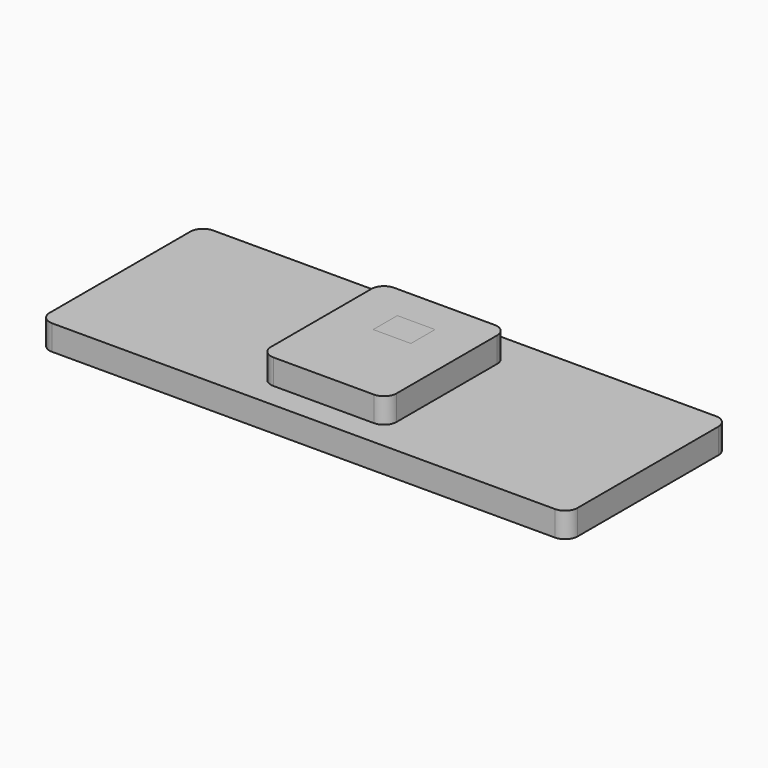
from build123d import *

# Parameters (mm, degrees)
F1_START = 2
F1_DEPTH = 1
F2_DEPTH = 3
F3_START = 2
F0_W     = 1.5
F0_H     = 1.2
F3_DEPTH = 2
F4_START = 3.5
F4_DEPTH = 0.5


# Not quite as in the source:
# - a feature names something its author has since deleted; it is built from what else it names


with BuildPart() as f1:
    # F0 (on Top) → F1 (new body)
    with BuildSketch(Plane.XY.offset(F1_START)):
        with BuildLine():
            Line((10, 4), (-10, 4))
            ThreePointArc((-10, 4), (-10.3535533906, 3.8535533906), (-10.5, 3.5))
            Line((-10.5, 3.5), (-10.5, -3.5))
            ThreePointArc((-10.5, -3.5), (-10.3535533906, -3.8535533906), (-10, -4))
            Line((-10, -4), (10, -4))
            ThreePointArc((10, -4), (10.3535533906, -3.8535533906), (10.5, -3.5))
            Line((10.5, -3.5), (10.5, 3.5))
            ThreePointArc((10.5, 3.5), (10.3535533906, 3.8535533906), (10, 4))
        make_face()
        with BuildLine():
            ThreePointArc((-7.9, 0.5), (-7.7535533906, 0.8535533906), (-7.4, 1))
            Line((-7.4, 1), (-5.9, 1))
            Line((-5.9, 1), (-5.9, -1))
            Line((-5.9, -1), (-7.4, -1))
            ThreePointArc((-7.4, -1), (-7.7535533906, -0.8535533906), (-7.9, -0.5))
            Line((-7.9, -0.5), (-7.9, 0.5))
        make_face(mode=Mode.SUBTRACT)
        with BuildLine():
            Line((-2, 3), (2, 3))
            ThreePointArc((2, 3), (2.3535533906, 2.8535533906), (2.5, 2.5))
            Line((2.5, 2.5), (2.5, -2.5))
            ThreePointArc((2.5, -2.5), (2.3535533906, -2.8535533906), (2, -3))
            Line((2, -3), (-2, -3))
            ThreePointArc((-2, -3), (-2.3535533906, -2.8535533906), (-2.5, -2.5))
            Line((-2.5, -2.5), (-2.5, 2.5))
            ThreePointArc((-2.5, 2.5), (-2.3535533906, 2.8535533906), (-2, 3))
        make_face(mode=Mode.SUBTRACT)
        with BuildLine():
            Line((5.9, -1), (5.9, 1))
            Line((5.9, 1), (7.4, 1))
            ThreePointArc((7.4, 1), (7.7535533906, 0.8535533906), (7.9, 0.5))
            Line((7.9, 0.5), (7.9, -0.5))
            ThreePointArc((7.9, -0.5), (7.7535533906, -0.8535533906), (7.4, -1))
            Line((7.4, -1), (5.9, -1))
        make_face(mode=Mode.SUBTRACT)
    extrude(amount=F1_DEPTH)

    # F0 (on Top) → F2 (join)
    with BuildSketch(Plane.XY):
        with BuildLine():
            Line((-5.9, 1), (-7.4, 1))
            ThreePointArc((-7.4, 1), (-7.7535533906, 0.8535533906), (-7.9, 0.5))
            Line((-7.9, 0.5), (-7.9, -0.5))
            ThreePointArc((-7.9, -0.5), (-7.7535533906, -0.8535533906), (-7.4, -1))
            Line((-7.4, -1), (-5.9, -1))
            Line((-5.9, -1), (-5.9, 1))
        make_face()
        with BuildLine():
            Line((7.4, 1), (5.9, 1))
            Line((5.9, 1), (5.9, -1))
            Line((5.9, -1), (7.4, -1))
            ThreePointArc((7.4, -1), (7.7535533906, -0.8535533906), (7.9, -0.5))
            Line((7.9, -0.5), (7.9, 0.5))
            ThreePointArc((7.9, 0.5), (7.7535533906, 0.8535533906), (7.4, 1))
        make_face()
    extrude(amount=F2_DEPTH)

    # F0 (on Top) → F3 (join)
    with BuildSketch(Plane.XY.offset(F3_START)):
        with BuildLine():
            ThreePointArc((2.5, 2.5), (2.3535533906, 2.8535533906), (2, 3))
            Line((2, 3), (-2, 3))
            ThreePointArc((-2, 3), (-2.3535533906, 2.8535533906), (-2.5, 2.5))
            Line((-2.5, 2.5), (-2.5, -2.5))
            ThreePointArc((-2.5, -2.5), (-2.3535533906, -2.8535533906), (-2, -3))
            Line((-2, -3), (2, -3))
            ThreePointArc((2, -3), (2.3535533906, -2.8535533906), (2.5, -2.5))
            Line((2.5, -2.5), (2.5, 2.5))
        make_face()
        with Locations((0, 1)):
            Rectangle(F0_W, F0_H, mode=Mode.SUBTRACT)
    extrude(amount=F3_DEPTH)


with BuildPart() as f4:
    # F0 (on Top) → F4 (new body)
    with BuildSketch(Plane.XY.offset(F4_START)):
        with Locations((0, 1)):
            Rectangle(F0_W, F0_H)
    extrude(amount=F4_DEPTH)


solid = Compound([f1.part, f4.part])
